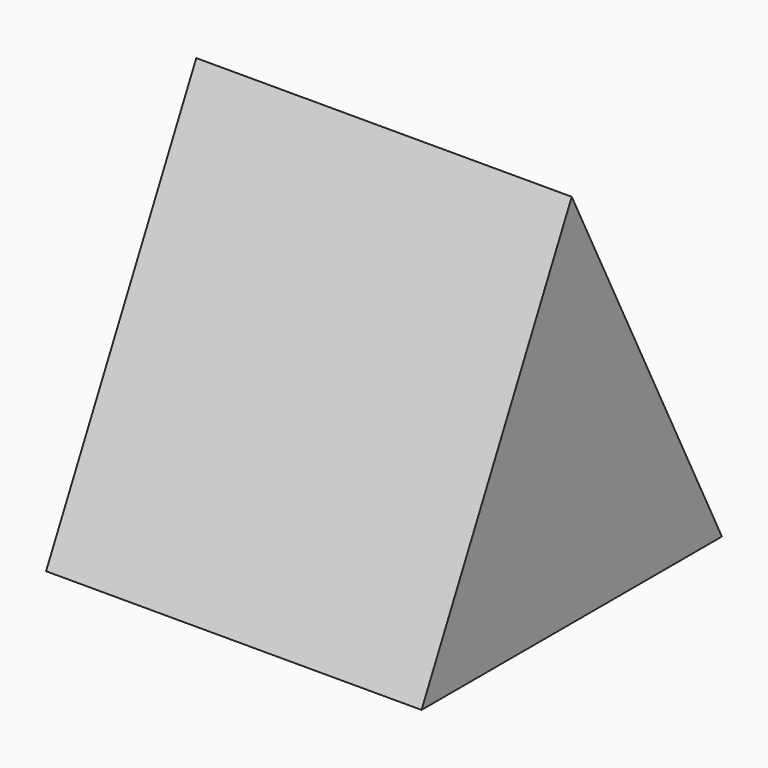
from build123d import *

# Parameters (mm, degrees)
F1_DEPTH = 25
F2_DEPTH = 25
F4_DEPTH = 25


# Not quite as in the source:
# - a feature of the source that left no trace in its solid (it failed there, or was rolled back) is left out


with BuildPart() as f1:
    # F0 (on Right) → F1 (new body)
    with BuildSketch(Plane.YZ):
        Polygon((-25, 0), (0, 0), (0, 50), align=None)
        Polygon((0, 50), (0, 0), (25, 0), align=None)
    extrude(amount=F1_DEPTH)

    # F2 (add): a face of the model
    f2_faces = [f1.faces().sort_by_distance(p)[0] for p in [
        (0, 0, 16.6666666667),
    ]]
    extrude(f2_faces, amount=F2_DEPTH)

    # F3 (on face) → F4 (cut)
    with BuildSketch(Plane(origin=(-25, 0, 0), x_dir=(0, -1, 0), z_dir=(-1, 0, 0))):
        Polygon((-13.9194109071, 5.4563577287), (0, 5.4563577287), (0, 42.9563577287), align=None)
        Polygon((0, 42.9563577287), (0, 5.4563577287), (13.9194109071, 5.4563577287), align=None)
    extrude(amount=-F4_DEPTH, mode=Mode.SUBTRACT)


solid = f1.part
